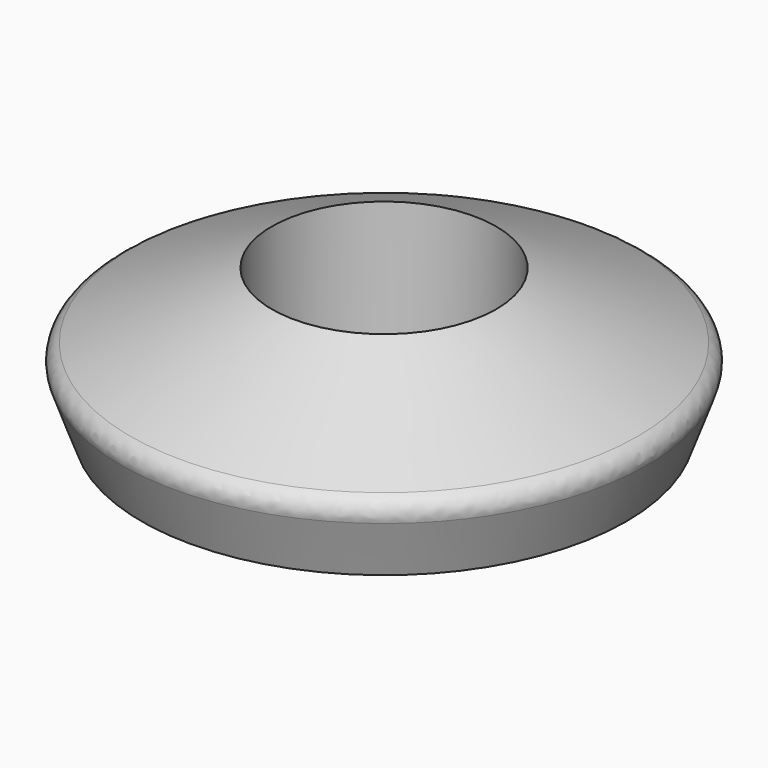
from build123d import *

# Parameters (mm, degrees)
F0_R          = 75
F1_DEPTH      = 50
F1_TAPER      = 65
F1_DEPTH_BACK = 20
F1_TAPER_BACK = 20
F2_R          = 5
F3_R          = 31.3436912466
F4_DEPTH      = 50
F4_DEPTH_BACK = 25


with BuildPart() as f1:
    # F0 (on Top) → F1 (new body, two sides)
    with BuildSketch(Plane.XY) as f1_sk:
        Circle(F0_R)
    extrude(amount=F1_DEPTH, taper=F1_TAPER)
    extrude(f1_sk.sketch, amount=-F1_DEPTH_BACK, taper=F1_TAPER_BACK)

    # F2
    f2_edges = [f1.edges().sort_by_distance(p)[0] for p in [
        (-75, 0, 0),
    ]]
    fillet(f2_edges, radius=F2_R)

    # F3 (on Top) → F4 (cut, two sides)
    with BuildSketch(Plane.XY) as f4_sk:
        Circle(F3_R)
    extrude(amount=F4_DEPTH, mode=Mode.SUBTRACT)
    extrude(f4_sk.sketch, amount=-F4_DEPTH_BACK, mode=Mode.SUBTRACT)


solid = f1.part
